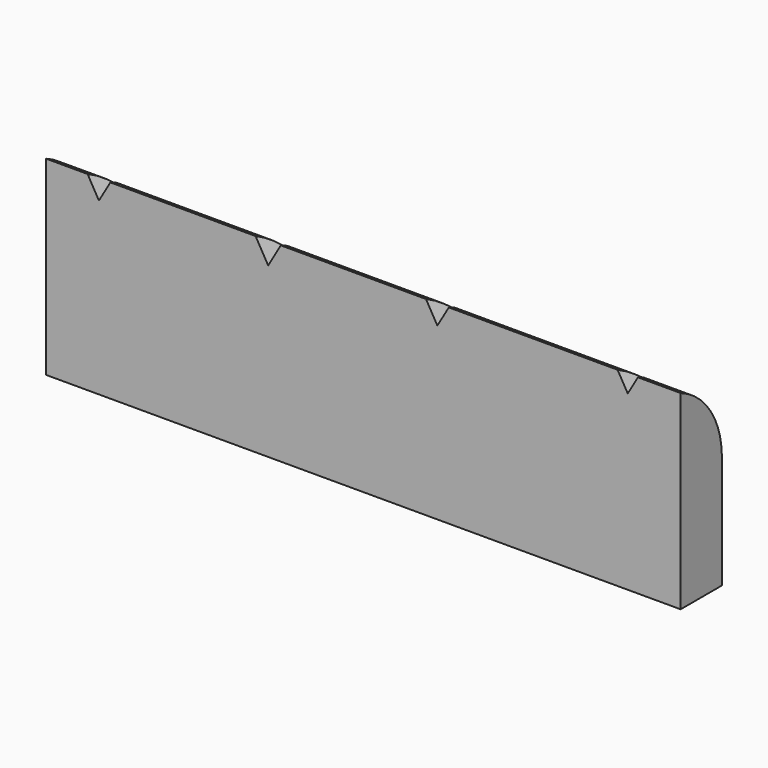
from build123d import *

# Parameters (mm, degrees)
F0_W        = 38.1
F0_H        = 3.0988
F1_DEPTH    = 11.43
F3_T1_DEPTH = 61.4886973558
F4_DEPTH    = 25.4


# Not quite as in the source:
# - a fillet or chamfer that OpenCascade refuses, or shapes differently, is made with other operations: its cross-section is extruded or revolved along the edge and cut away or added


with BuildPart() as f1:
    # F0 (on Top) → F1 (new body)
    with BuildSketch(Plane.XY):
        with Locations((0, 1.5494)):
            Rectangle(F0_W, F0_H)
    extrude(amount=F1_DEPTH)

    # F3: fillet of radius 5.08 on 1 edges, made by hand

    # F3_s2 → F3_t1 (cut)
    with BuildSketch(Plane.YZ.offset(-30.7443486779)):
        with BuildLine():
            ThreePointArc((3.0988, 6.7522605288), (2.2538263281, 9.5577822272), (0, 11.43))
            Line((0, 11.43), (3.0988, 11.43))
            Line((3.0988, 11.43), (3.0988, 6.7522605288))
        make_face()
    extrude(amount=F3_T1_DEPTH, mode=Mode.SUBTRACT)

    # F2 (on face) → F4 (cut)
    with BuildSketch(Plane.XZ):
        Polygon((-15.875, 10.2462954744), (-15.1915878735, 11.43), (-16.5584121265, 11.43), align=None)
        Polygon((-4.9582643893, 11.43), (-6.4717356107, 11.43), (-5.715, 10.1192954744), align=None)
        Polygon((5.1284121265, 11.43), (3.7615878735, 11.43), (4.445, 10.2462954744), align=None)
        Polygon((16.4850886423, 11.43), (15.2649113577, 11.43), (15.875, 10.3732954744), align=None)
    extrude(amount=-F4_DEPTH, mode=Mode.SUBTRACT)


solid = f1.part
